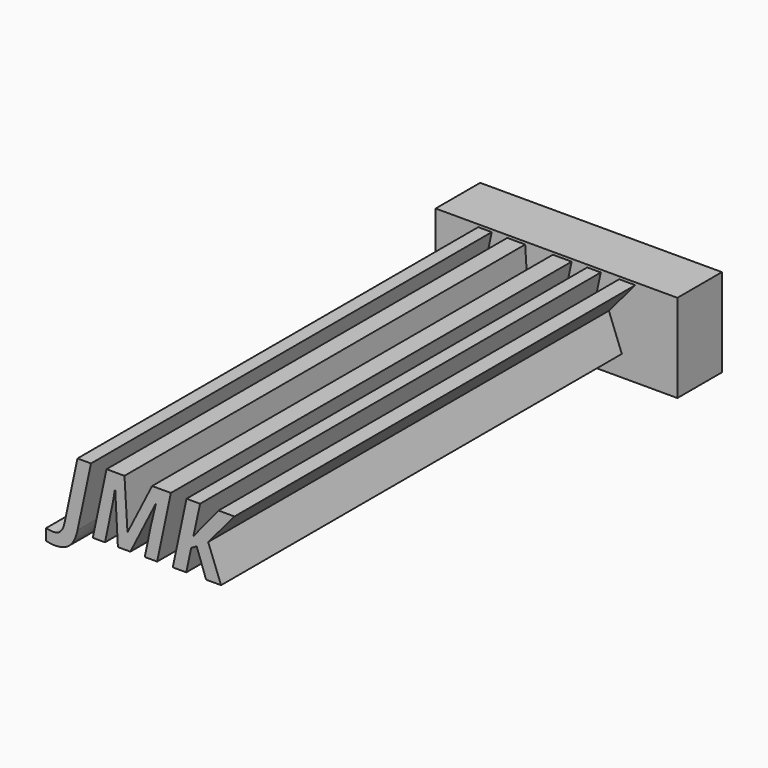
from build123d import *

# Parameters (mm, degrees)
F0_W         = 110.3363707662
F0_H         = 40.2815341949
F1_DEPTH     = 25.4
F2_TEXT_SIZE = 41.4798404866
F3_DEPTH     = 25.4
F4_DEPTH     = 25.4
F5_DEPTH     = 254


# Not quite as in the source:
# - Text() gives the source's letters only with a copy of the font that has no kerning and outlines rounded to 1/6400 em; it was checked with that copy


with BuildPart() as f1:
    # F0 (on Front) → F1 (new body)
    with BuildSketch(Plane.XZ):
        with Locations((55.1681853831, 20.1407670975)):
            Rectangle(F0_W, F0_H)
    extrude(amount=F1_DEPTH)

    # F2 (on Front) → F3 (join)
    with BuildSketch(Plane.XZ):
        with Locations((11.6297157947, 9.494274389)):
            Text('JMK', F2_TEXT_SIZE, font='Open Sans', font_style=FontStyle.BOLDITALIC, text_align=(TextAlign.LEFT, TextAlign.BOTTOM))
    extrude(amount=F3_DEPTH)

    # F2 (on Front) → F4 (join)
    with BuildSketch(Plane.XZ):
        with Locations((11.6297157947, 9.494274389)):
            Text('JMK', F2_TEXT_SIZE, font='Open Sans', font_style=FontStyle.BOLDITALIC, text_align=(TextAlign.LEFT, TextAlign.BOTTOM))
    extrude(amount=F4_DEPTH)

    # F2 (on Front) → F5 (join)
    with BuildSketch(Plane.XZ):
        with Locations((11.6297157947, 9.494274389)):
            Text('JMK', F2_TEXT_SIZE, font='Open Sans', font_style=FontStyle.BOLDITALIC, text_align=(TextAlign.LEFT, TextAlign.BOTTOM))
    extrude(amount=F5_DEPTH)


solid = f1.part
